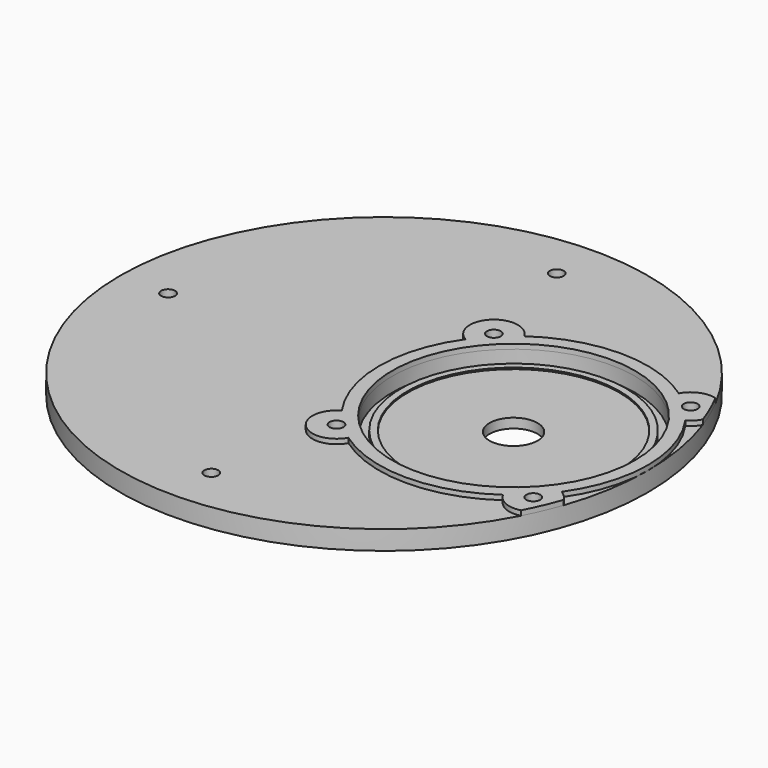
from build123d import *

# Parameters (mm, degrees)
F0_R      = 55
F1_DEPTH  = 4
F2_R      = 22.1
F3_DEPTH  = 2
F4_R      = 25.3
F4_R_2    = 22.1
F5_DEPTH  = 1.5
F6_R      = 25.3
F6_R_2    = 23.5
F7_DEPTH  = 1.5
F8_DEPTH  = 0.2
F9_R      = 28
F9_R_2    = 25.3
F10_DEPTH = 1
F11_R     = 5
F12_DEPTH = 25
F14_DEPTH = 1
F15_R     = 1.45
F16_DEPTH = 25
F17_R     = 1.45
F18_DEPTH = 25


with BuildPart() as f1:
    # F0 (on Top) → F1 (new body)
    with BuildSketch(Plane.XY):
        Circle(F0_R)
    extrude(amount=F1_DEPTH)

    # F2 (on face) → F3 (cut)
    with BuildSketch(Plane.XY.offset(4)):
        with Locations((27, 0)):
            Circle(F2_R)
    extrude(amount=-F3_DEPTH, mode=Mode.SUBTRACT)

    # F4 (on face) → F5 (cut)
    with BuildSketch(Plane.XY.offset(4)):
        with Locations((27, 0)):
            Circle(F4_R)
        with Locations((27, 0)):
            Circle(F4_R_2, mode=Mode.SUBTRACT)
    extrude(amount=-F5_DEPTH, mode=Mode.SUBTRACT)

    # F6 (on face) → F7 (cut)
    with BuildSketch(Plane.XY.offset(2.5)):
        with Locations((27, 0)):
            Circle(F6_R)
        with Locations((27, 0)):
            Circle(F6_R_2, mode=Mode.SUBTRACT)
    extrude(amount=-F7_DEPTH, mode=Mode.SUBTRACT)

    # F8 (cut): a face of the model
    f8_faces = [f1.faces().sort_by_distance(p)[0] for p in [
        (4.1646803743, 0, 2.5),
    ]]
    extrude(f8_faces, amount=-F8_DEPTH, mode=Mode.SUBTRACT)

    # F9 (on face) → F10 (join)
    with BuildSketch(Plane.XY.offset(4)):
        with Locations((27, 0)):
            Circle(F9_R)
        with Locations((27, 0)):
            Circle(F9_R_2, mode=Mode.SUBTRACT)
    extrude(amount=F10_DEPTH)

    # F11 (on face) → F12 (cut)
    with BuildSketch(Plane.XY.offset(2)):
        with Locations((27, 0)):
            Circle(F11_R)
    extrude(amount=-F12_DEPTH, mode=Mode.SUBTRACT)

    # F13 (on face) → F14 (join)
    with BuildSketch(Plane.XY.offset(4)):
        with BuildLine():
            ThreePointArc((10.8848586854, -22.8976466129), (7.2010101268, -19.7989898732), (4.1023533871, -16.1151413146))
            ThreePointArc((4.1023533871, -16.1151413146), (2.9583694397, -24.0416305603), (10.8848586854, -22.8976466129))
        make_face()
        with BuildLine():
            ThreePointArc((10.8848586854, 22.8976466129), (2.9583694397, 24.0416305603), (4.1023533871, 16.1151413146))
            ThreePointArc((4.1023533871, 16.1151413146), (7.2010101268, 19.7989898732), (10.8848586854, 22.8976466129))
        make_face()
        with BuildLine():
            ThreePointArc((49.8976466129, -16.1151413146), (46.7989898732, -19.7989898732), (43.1151413146, -22.8976466129))
            ThreePointArc((43.1151413146, -22.8976466129), (45.5447053375, -25.105329645), (48.8197581332, -25.3304404978))
            ThreePointArc((48.8197581332, -25.3304404978), (50.4964850216, -21.7969034605), (51.917853321, -18.1531404043))
            ThreePointArc((51.917853321, -18.1531404043), (51.0570972643, -16.9860974117), (49.8976466129, -16.1151413146))
        make_face()
        with BuildLine():
            ThreePointArc((48.8197581332, 25.3304404978), (45.5447053375, 25.105329645), (43.1151413146, 22.8976466129))
            ThreePointArc((43.1151413146, 22.8976466129), (46.7989898732, 19.7989898732), (49.8976466129, 16.1151413146))
            ThreePointArc((49.8976466129, 16.1151413146), (51.0570972643, 16.9860974117), (51.917853321, 18.1531404043))
            ThreePointArc((51.917853321, 18.1531404043), (50.4964850216, 21.7969034605), (48.8197581332, 25.3304404978))
        make_face()
    extrude(amount=F14_DEPTH)

    # F15 (on face) → F16 (cut)
    with BuildSketch(Plane.XY.offset(5)):
        with Locations((6.4939033456, 20.5060966544)):
            Circle(F15_R)
        with Locations((47.5060966544, 20.5060966544)):
            Circle(F15_R)
        with Locations((47.5060966544, -20.5060966544)):
            Circle(F15_R)
        with Locations((6.4939033456, -20.5060966544)):
            Circle(F15_R)
    extrude(amount=-F16_DEPTH, mode=Mode.SUBTRACT)

    # F17 (on face) → F18 (cut)
    with BuildSketch(Plane.XY.offset(4)):
        with Locations((0, 45)):
            Circle(F17_R)
        with Locations((-45, 0)):
            Circle(F17_R)
        with Locations((0, -45)):
            Circle(F17_R)
    extrude(amount=-F18_DEPTH, mode=Mode.SUBTRACT)


solid = f1.part
